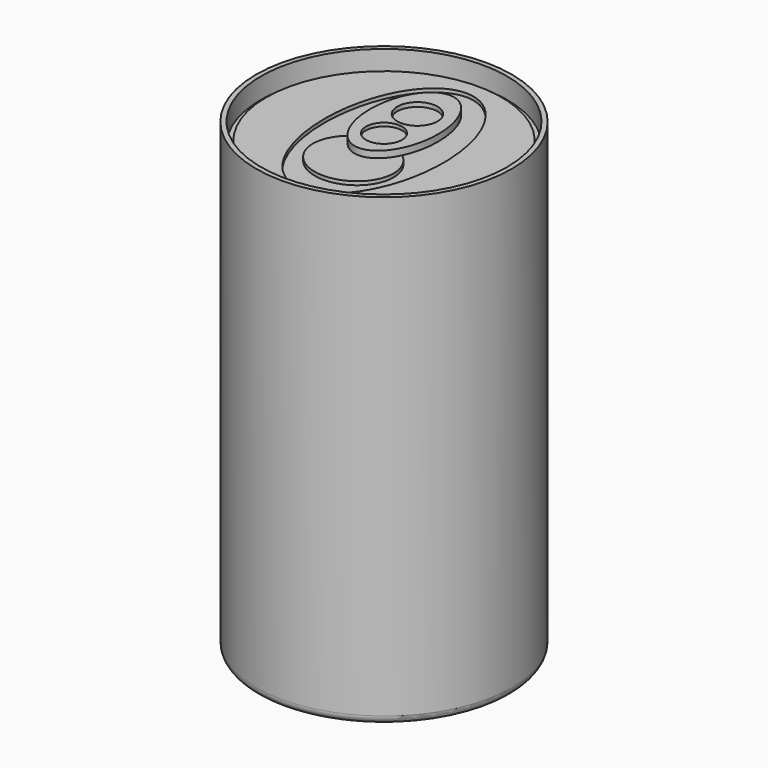
from build123d import *

# Parameters (mm, degrees)
F0_R      = 75.279024749
F1_DEPTH  = 104
F2_DEPTH  = 131
F3_DEPTH  = 39
F4_R      = 72.4752953546
F5_DEPTH  = 12.2
F6_R      = 69.3178574883
F7_DEPTH  = 2.3
F10_DEPTH = 2.1
F12_DEPTH = 3.9
F14_DEPTH = 2.4
F15_R     = 11.830371828
F16_DEPTH = 2.5
F15_R_2   = 10.6100179521
F17_DEPTH = 2
F18_R     = 57.314692
F19_DEPTH = 8.7
F20_R     = 5


with BuildPart() as f1:
    # F0 (on Top) → F1 (new body)
    with BuildSketch(Plane.XY):
        Circle(F0_R)
    extrude(amount=F1_DEPTH)

    # F2 (add): a face of the model
    f2_faces = [f1.faces().sort_by_distance(p)[0] for p in [
        (0, 0, 0),
    ]]
    extrude(f2_faces, amount=F2_DEPTH)

    # F3 (add): a face of the model
    f3_faces = [f1.faces().sort_by_distance(p)[0] for p in [
        (0, 0, 104),
    ]]
    extrude(f3_faces, amount=F3_DEPTH)

    # F4 (on face) → F5 (cut)
    with BuildSketch(Plane.XY.offset(143)):
        Circle(F4_R)
    extrude(amount=-F5_DEPTH, mode=Mode.SUBTRACT)

    # F6 (on face) → F7 (join)
    with BuildSketch(Plane.XY.offset(130.8)):
        Circle(F6_R)
    extrude(amount=F7_DEPTH)

    # F9 (on face) → F10 (cut)
    with BuildSketch(Plane.XY.offset(133.1)):
        with BuildLine():
            add(Edge.make_bspline(
                [(0, 60.7038661838), (-60.7799193233, 60.7038661838), (-30.3899596616, -30.3519330919), (0, -121.4077323675), (30.3899596616, -30.3519330919), (60.7799193233, 60.7038661838), (0, 60.7038661838)],
                knots=[0, 0, 0, 2.0943951024, 2.0943951024, 4.1887902048, 4.1887902048, 6.2831853072, 6.2831853072, 6.2831853072], degree=2, weights=[1, 0.5, 1, 0.5, 1, 0.5, 1]))
        make_face()
    extrude(amount=-F10_DEPTH, mode=Mode.SUBTRACT)

    # F18 (on face) → F19 (cut)
    with BuildSketch(Plane(origin=(0, 0, -131), x_dir=(1, 0, 0), z_dir=(0, 0, -1))):
        Circle(F18_R)
    extrude(amount=-F19_DEPTH, mode=Mode.SUBTRACT)

    # F20
    f20_edges = [f1.edges().sort_by_distance(p)[0] for p in [
        (-75.279025, 0, -131),
        (-57.314692, 0, -131),
    ]]
    fillet(f20_edges, radius=F20_R)


with BuildPart() as f12:
    # F11 (on face) → F12 (new body)
    with BuildSketch(Plane.XY.offset(133.1)):
        with BuildLine():
            add(Edge.make_bspline(
                [(0, 48.477794975), (-34.7240676564, 48.477794975), (-17.3620338282, -1.8481253646), (0, -52.1740457043), (17.3620338282, -1.8481253646), (34.7240676564, 48.477794975), (0, 48.477794975)],
                knots=[0, 0, 0, 2.0943951024, 2.0943951024, 4.1887902048, 4.1887902048, 6.2831853072, 6.2831853072, 6.2831853072], degree=2, weights=[1, 0.5, 1, 0.5, 1, 0.5, 1]))
        make_face()
    extrude(amount=F12_DEPTH)

    # F13 (on face) → F14 (join)
    with BuildSketch(Plane.XY.offset(133.1)):
        with BuildLine():
            add(Edge.make_bspline(
                [(23.7413235009, -22.6040165871), (23.7413235009, 15.470016879), (-11.8706617504, -3.5669998541), (-47.4826470017, -22.6040165871), (-11.8706617504, -41.6410333202), (23.7413235009, -60.6780500532), (23.7413235009, -22.6040165871)],
                knots=[0, 0, 0, 2.0943951024, 2.0943951024, 4.1887902048, 4.1887902048, 6.2831853072, 6.2831853072, 6.2831853072], degree=2, weights=[1, 0.5, 1, 0.5, 1, 0.5, 1]))
        make_face()
    extrude(amount=-F14_DEPTH)

    # F15 (on face) → F16 (cut)
    with BuildSketch(Plane.XY.offset(137)):
        with Locations((0, 24.5943088084)):
            Circle(F15_R)
    extrude(amount=-F16_DEPTH, mode=Mode.SUBTRACT)

    # F15 (on face) → F17 (cut)
    with BuildSketch(Plane.XY.offset(137)):
        Circle(F15_R_2)
    extrude(amount=-F17_DEPTH, mode=Mode.SUBTRACT)


solid = Compound([f1.part, f12.part])
